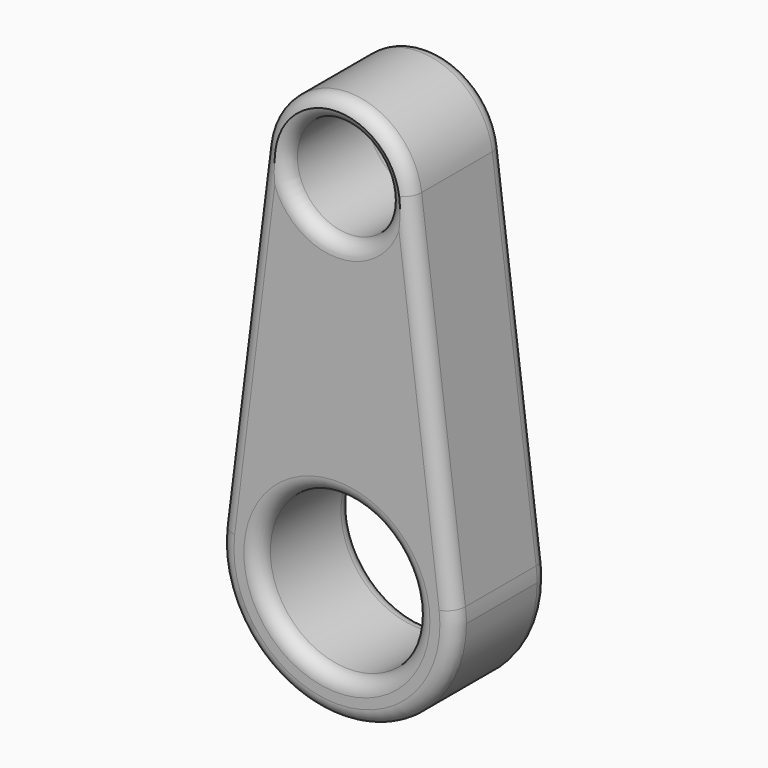
from build123d import *

# Parameters (mm, degrees)
F0_R         = 26.615795876
F0_R_2       = 17.4268543136
F1_DEPTH     = 40
F2_T1_DEPTH  = 120
F2_T3_DEPTH  = 120
F2_T14_ANGLE = 165.7499673022
F2_T16_ANGLE = 165.7499673022
F2_T18_ANGLE = 194.2500326978
F2_T20_ANGLE = 194.2500326978


# Not quite as in the source:
# - a fillet or chamfer that OpenCascade refuses, or shapes differently, is made with other operations: its cross-section is extruded or revolved along the edge and cut away or added


with BuildPart() as f1:
    # F0 (on Front) → F1 (new body)
    with BuildSketch(Plane.XZ):
        with BuildLine():
            ThreePointArc((-39.6911150685, -15.3067131157), (-2.4854976623, -60.1908065831), (40, -20.2681024992))
            ThreePointArc((40, -20.2681024992), (39.9227040839, -17.782604837), (39.6911150685, -15.3067131157))
            ThreePointArc((39.6911150685, -15.3067131157), (0, 19.7318975008), (-39.6911150685, -15.3067131157))
        make_face()
        with Locations((0, -20.2681024992)):
            Circle(F0_R, mode=Mode.SUBTRACT)
        with BuildLine():
            ThreePointArc((-39.6911150685, -15.3067131157), (0, 19.7318975008), (39.6911150685, -15.3067131157))
            Line((39.6911150685, -15.3067131157), (24.8069469178, 103.76663209))
            ThreePointArc((24.8069469178, 103.76663209), (24.9516900524, 102.2191997641), (25, 100.6657637252))
            ThreePointArc((25, 100.6657637252), (-1.5534360389, 75.7140736728), (-24.8069469178, 103.76663209))
            Line((-24.8069469178, 103.76663209), (-39.6911150685, -15.3067131157))
        make_face()
        with BuildLine():
            ThreePointArc((25, 100.6657637252), (24.9516900524, 102.2191997641), (24.8069469178, 103.76663209))
            ThreePointArc((24.8069469178, 103.76663209), (0, 125.6657637252), (-24.8069469178, 103.76663209))
            ThreePointArc((-24.8069469178, 103.76663209), (-1.5534360389, 75.7140736728), (25, 100.6657637252))
        make_face()
        with Locations((0, 100.6657637252)):
            Circle(F0_R_2, mode=Mode.SUBTRACT)
    extrude(amount=F1_DEPTH)

    # F2: fillet of radius 5 on 8 edges, made by hand

    # F2_s2 → F2_t1 (cut)
    with BuildSketch(Plane(origin=(2.4945356922, 0, -19.9562855377), x_dir=(0, 1, 0), z_dir=(-0.1240347346, 0, 0.9922778767))):
        with BuildLine():
            ThreePointArc((-5, -37.4860512859), (-1.4644660941, -36.0215851918), (0, -32.4860512859))
            Line((0, -32.4860512859), (0, -37.4860512859))
            Line((0, -37.4860512859), (-5, -37.4860512859))
        make_face()
        with BuildLine():
            ThreePointArc((-35, -37.4860512859), (-38.5355339059, -36.0215851918), (-40, -32.4860512859))
            Line((-40, -32.4860512859), (-40, -37.4860512859))
            Line((-40, -37.4860512859), (-35, -37.4860512859))
        make_face()
    extrude(amount=F2_T1_DEPTH, mode=Mode.SUBTRACT)

    # F2_s4 → F2_t3 (cut)
    with BuildSketch(Plane(origin=(12.3896324585, 0, 99.1170596679), x_dir=(0, 1, 0), z_dir=(-0.1240347346, 0, -0.9922778767))):
        with BuildLine():
            ThreePointArc((-35, -37.4860512859), (-38.5355339059, -36.0215851918), (-40, -32.4860512859))
            Line((-40, -32.4860512859), (-40, -37.4860512859))
            Line((-40, -37.4860512859), (-35, -37.4860512859))
        make_face()
        with BuildLine():
            ThreePointArc((-5, -37.4860512859), (-1.4644660941, -36.0215851918), (0, -32.4860512859))
            Line((0, -32.4860512859), (0, -37.4860512859))
            Line((0, -37.4860512859), (-5, -37.4860512859))
        make_face()
    extrude(amount=F2_T3_DEPTH, mode=Mode.SUBTRACT)

    # F2_s5 → F2_t6 (revolve, cut)
    with BuildSketch(Plane.XY.offset(100.6657637252)):
        with BuildLine():
            ThreePointArc((17.4268543136, -35), (18.8913204077, -38.5355339059), (22.4268543136, -40))
            Line((22.4268543136, -40), (17.4268543136, -40))
            Line((17.4268543136, -40), (17.4268543136, -35))
        make_face()
    revolve(axis=Axis((0, -40, 100.6657637252), (0, -1, 0)), mode=Mode.SUBTRACT)

    # F2_s7 → F2_t8 (revolve, cut)
    with BuildSketch(Plane.XY.offset(-20.2681024992)):
        with BuildLine():
            ThreePointArc((26.615795876, -35), (28.0802619701, -38.5355339059), (31.615795876, -40))
            Line((31.615795876, -40), (26.615795876, -40))
            Line((26.615795876, -40), (26.615795876, -35))
        make_face()
    revolve(axis=Axis((0, -40, -20.2681024992), (0, -1, 0)), mode=Mode.SUBTRACT)

    # F2_s9 → F2_t10 (revolve, cut)
    with BuildSketch(Plane.XY.offset(-20.2681024992)):
        with BuildLine():
            ThreePointArc((26.615795876, -5), (28.0802619701, -1.4644660941), (31.615795876, 0))
            Line((31.615795876, 0), (26.615795876, 0))
            Line((26.615795876, 0), (26.615795876, -5))
        make_face()
    revolve(axis=Axis((0, 0, -20.2681024992), (0, -1, 0)), mode=Mode.SUBTRACT)

    # F2_s11 → F2_t12 (revolve, cut)
    with BuildSketch(Plane.XY.offset(100.6657637252)):
        with BuildLine():
            ThreePointArc((17.4268543136, -5), (18.8913204077, -1.4644660941), (22.4268543136, 0))
            Line((22.4268543136, 0), (17.4268543136, 0))
            Line((17.4268543136, 0), (17.4268543136, -5))
        make_face()
    revolve(axis=Axis((0, 0, 100.6657637252), (0, -1, 0)), mode=Mode.SUBTRACT)

    # F2_s13 → F2_t14 (revolve, cut)
    with BuildSketch(Plane(origin=(-12.3896324585, 0, 99.1170596679), x_dir=(0, 1, 0), z_dir=(0.1240347346, 0, -0.9922778767))):
        with BuildLine():
            ThreePointArc((-5, 37.4860512859), (-1.4644660941, 36.0215851918), (0, 32.4860512859))
            Line((0, 32.4860512859), (0, 37.4860512859))
            Line((0, 37.4860512859), (-5, 37.4860512859))
        make_face()
    revolve(axis=Axis((0, 0, 100.6657637252), (0, -1, 0)), revolution_arc=F2_T14_ANGLE, mode=Mode.SUBTRACT)

    # F2_s15 → F2_t16 (revolve, cut)
    with BuildSketch(Plane(origin=(-12.3896324585, 0, 99.1170596679), x_dir=(0, 1, 0), z_dir=(0.1240347346, 0, -0.9922778767))):
        with BuildLine():
            ThreePointArc((-35, 37.4860512859), (-38.5355339059, 36.0215851918), (-40, 32.4860512859))
            Line((-40, 32.4860512859), (-40, 37.4860512859))
            Line((-40, 37.4860512859), (-35, 37.4860512859))
        make_face()
    revolve(axis=Axis((0, -40, 100.6657637252), (0, -1, 0)), revolution_arc=F2_T16_ANGLE, mode=Mode.SUBTRACT)

    # F2_s17 → F2_t18 (revolve, cut)
    with BuildSketch(Plane(origin=(-2.4945356922, 0, -19.9562855377), x_dir=(0, 1, 0), z_dir=(0.1240347346, 0, 0.9922778767))):
        with BuildLine():
            ThreePointArc((-35, 37.4860512859), (-38.5355339059, 36.0215851918), (-40, 32.4860512859))
            Line((-40, 32.4860512859), (-40, 37.4860512859))
            Line((-40, 37.4860512859), (-35, 37.4860512859))
        make_face()
    revolve(axis=Axis((0, -40, -20.2681024992), (0, -1, 0)), revolution_arc=F2_T18_ANGLE, mode=Mode.SUBTRACT)

    # F2_s19 → F2_t20 (revolve, cut)
    with BuildSketch(Plane(origin=(-2.4945356922, 0, -19.9562855377), x_dir=(0, 1, 0), z_dir=(0.1240347346, 0, 0.9922778767))):
        with BuildLine():
            ThreePointArc((-5, 37.4860512859), (-1.4644660941, 36.0215851918), (0, 32.4860512859))
            Line((0, 32.4860512859), (0, 37.4860512859))
            Line((0, 37.4860512859), (-5, 37.4860512859))
        make_face()
    revolve(axis=Axis((0, 0, -20.2681024992), (0, -1, 0)), revolution_arc=F2_T20_ANGLE, mode=Mode.SUBTRACT)


solid = f1.part
